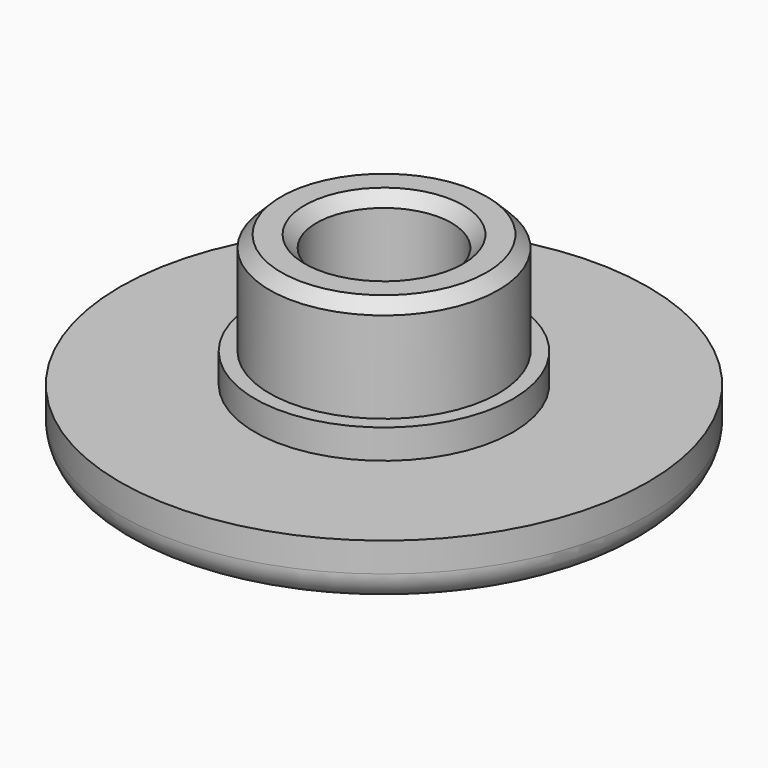
from build123d import *

# Parameters (mm, degrees)
F0_R     = 9
F0_R_2   = 4.4
F1_DEPTH = 2
F0_R_3   = 2.3
F0_R_4   = 3.9
F2_DEPTH = 3
F3_DEPTH = 6.5
F4_R     = 1
F5_SIZE  = 0.4


with BuildPart() as f1:
    # F0 (on Top) → F1 (new body)
    with BuildSketch(Plane.XY):
        Circle(F0_R)
        Circle(F0_R_2, mode=Mode.SUBTRACT)
    extrude(amount=F1_DEPTH)

    # F0 (on Top) → F2 (join)
    with BuildSketch(Plane.XY):
        Circle(F0_R_2)
        Circle(F0_R_4, mode=Mode.SUBTRACT)
    extrude(amount=F2_DEPTH)

    # F0 (on Top) → F3 (join)
    with BuildSketch(Plane.XY):
        Circle(F0_R_4)
        Circle(F0_R_3, mode=Mode.SUBTRACT)
    extrude(amount=F3_DEPTH)

    # F4
    f4_edges = [f1.edges().sort_by_distance(p)[0] for p in [
        (-9, 0, 0),
    ]]
    fillet(f4_edges, radius=F4_R)

    # F5
    f5_edges = [f1.edges().sort_by_distance(p)[0] for p in [
        (-3.9, 0, 6.5),
        (-2.3, 0, 6.5),
    ]]
    chamfer(f5_edges, length=F5_SIZE)


with BuildPart() as f1b:
    # F0 (on Top) → F1, piece 2 (new body)
    with BuildSketch(Plane.XY):
        Circle(F0_R_3)
    extrude(amount=F1_DEPTH)


solid = Compound([f1.part, f1b.part])
